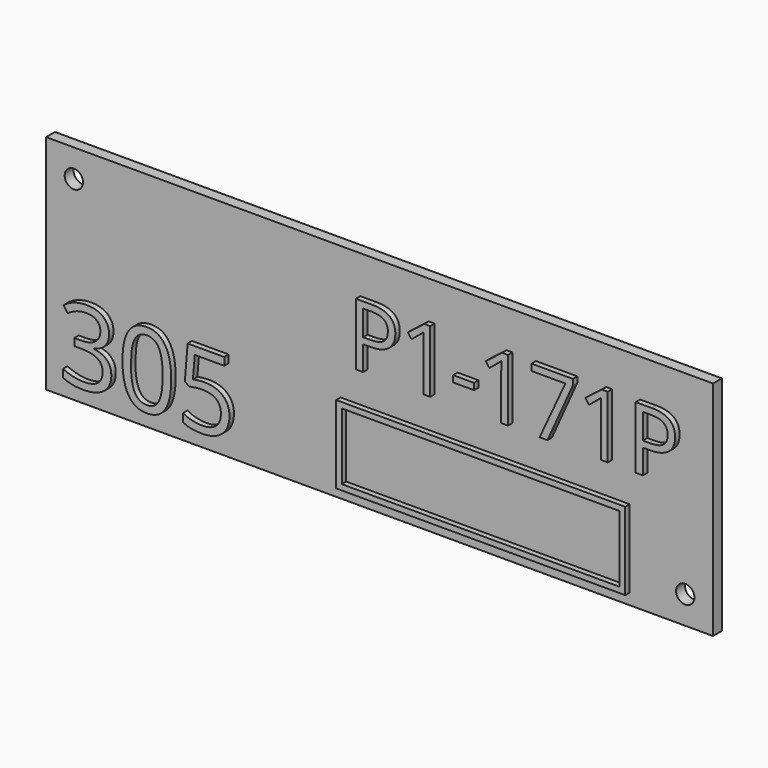
from build123d import *

# Parameters (mm, degrees)
F0_W         = 120
F0_H         = 40
F1_DEPTH     = 2
F3_D         = 3.3
F4_TEXT_SIZE = 15.681149951
F5_DEPTH     = 1
F6_TEXT_SIZE = 18.5776487663
F7_DEPTH     = 1
F8_W         = 52
F8_H         = 14
F8_W_2       = 49.99999962
F8_H_2       = 11.99999962
F9_DEPTH     = 1


# Not quite as in the source:
# - Text() gives the source's letters only with a copy of the font that has no kerning and outlines rounded to 1/6400 em; it was checked with that copy


with BuildPart() as f1:
    # F0 (on Front) → F1 (new body)
    with BuildSketch(Plane.XZ):
        Rectangle(F0_W, F0_H)
    extrude(amount=F1_DEPTH)

    # F3 (through all)
    with Locations(Plane.XZ.offset(2)):
        with Locations((-55, 15), (55, -15)):
            Hole(F3_D / 2)

    # F4 (on face) → F5 (join)
    with BuildSketch(Plane.XZ.offset(2)):
        with Locations((-5, 2)):
            Text('P1-171P', F4_TEXT_SIZE, font='Open Sans', text_align=(TextAlign.LEFT, TextAlign.BOTTOM))
    extrude(amount=F5_DEPTH)

    # F6 (on face) → F7 (join)
    with BuildSketch(Plane.XZ.offset(2)):
        with Locations((-57, -17)):
            Text('305', F6_TEXT_SIZE, font='Open Sans', text_align=(TextAlign.LEFT, TextAlign.BOTTOM))
    extrude(amount=F7_DEPTH)

    # F8 (on face) → F9 (join)
    with BuildSketch(Plane.XZ.offset(2)):
        with Locations((19, -11)):
            Rectangle(F8_W, F8_H)
        with Locations((19, -11)):
            Rectangle(F8_W_2, F8_H_2, mode=Mode.SUBTRACT)
    extrude(amount=F9_DEPTH)


solid = f1.part
